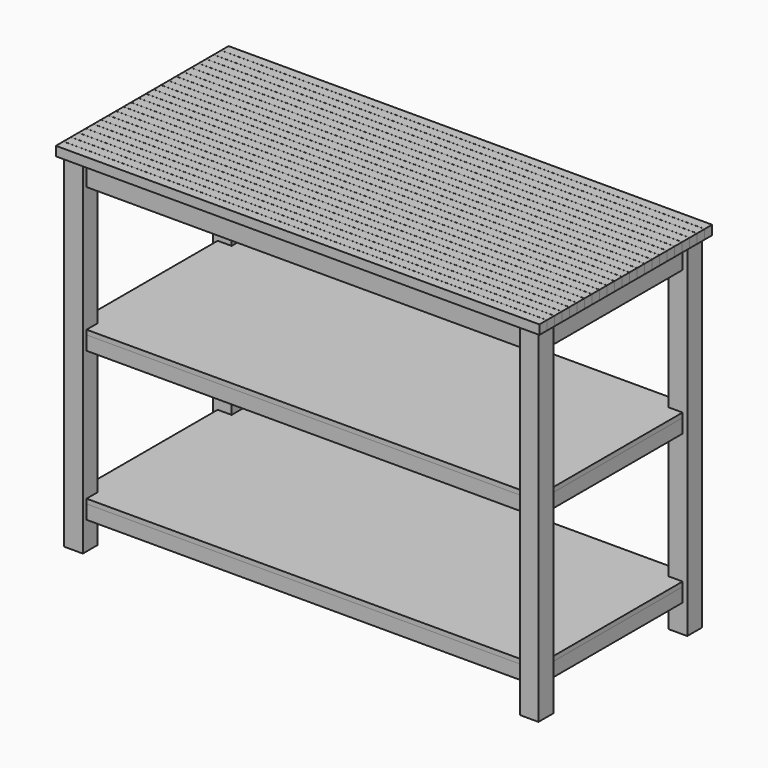
from build123d import *

# Parameters (mm, degrees)
F0_W      = 50.8
F0_H      = 50.8
F1_DEPTH  = 939.8
F2_W      = 1193.8
F2_H      = 25.4
F3_DEPTH  = 63.5
F2_W_2    = 25.4
F2_H_2    = 457.2
F5_W      = 1270
F5_H      = 533.4
F5_W_2    = 1219.2
F5_H_2    = 482.6
F6_DEPTH  = 38.1
F7_W      = 1270
F7_H      = 533.4
F8_DEPTH  = 12.7
F10_W     = 1270
F10_H     = 533.4
F10_W_2   = 1219.2
F10_H_2   = 482.6
F11_DEPTH = 38.1
F13_W     = 1320.8
F13_H     = 25.4
F14_DEPTH = 25.4
F12_W     = 1219.2
F12_H     = 482.6
F15_DEPTH = 12.7


# Not quite as in the source:
# - ends of sketch curves that miss each other by under 0.0002 mm in the source are joined


with BuildPart() as f1:
    # F0 (on Top) → F1 (new body)
    with BuildSketch(Plane.XY):
        with Locations((25.4, 25.4)):
            Rectangle(F0_W, F0_H)
    extrude(amount=F1_DEPTH)


with BuildPart() as f1b:
    # F0 (on Top) → F1, piece 2 (new body)
    with BuildSketch(Plane.XY):
        with Locations((25.4, 533.4)):
            Rectangle(F0_W, F0_H)
    extrude(amount=F1_DEPTH)


with BuildPart() as f1c:
    # F0 (on Top) → F1, piece 3 (new body)
    with BuildSketch(Plane.XY):
        with Locations((1270, 25.4)):
            Rectangle(F0_W, F0_H)
    extrude(amount=F1_DEPTH)


with BuildPart() as f1d:
    # F0 (on Top) → F1, piece 4 (new body)
    with BuildSketch(Plane.XY):
        with Locations((1270, 533.4)):
            Rectangle(F0_W, F0_H)
    extrude(amount=F1_DEPTH)


with BuildPart() as f3:
    # F2 (on face) → F3 (new body)
    with BuildSketch(Plane.XY.offset(939.8)):
        with Locations((647.7, 533.4)):
            Rectangle(F2_W, F2_H)
    extrude(amount=-F3_DEPTH)


with BuildPart() as f3b:
    # F2 (on face) → F3, piece 2 (new body)
    with BuildSketch(Plane.XY.offset(939.8)):
        with Locations((647.7, 25.4)):
            Rectangle(F2_W, F2_H)
    extrude(amount=-F3_DEPTH)


with BuildPart() as f3c:
    # F2 (on face) → F3, piece 3 (new body)
    with BuildSketch(Plane.XY.offset(939.8)):
        with Locations((25.4, 279.4)):
            Rectangle(F2_W_2, F2_H_2)
    extrude(amount=-F3_DEPTH)


with BuildPart() as f3d:
    # F2 (on face) → F3, piece 4 (new body)
    with BuildSketch(Plane.XY.offset(939.8)):
        with Locations((1270, 279.4)):
            Rectangle(F2_W_2, F2_H_2)
    extrude(amount=-F3_DEPTH)


with BuildPart() as f6:
    # F5 (on offset) → F6 (new body)
    with BuildSketch(Plane.XY.offset(76.2)):
        with Locations((647.7, 279.4)):
            Rectangle(F5_W, F5_H)
        with Locations((647.7, 279.4)):
            Rectangle(F5_W_2, F5_H_2, mode=Mode.SUBTRACT)
    extrude(amount=F6_DEPTH)


with BuildPart() as f8:
    # F7 (on face) → F8 (new body)
    with BuildSketch(Plane.XY.offset(114.3)):
        with Locations((647.7, 279.4)):
            Rectangle(F7_W, F7_H)
    extrude(amount=F8_DEPTH)


with BuildPart() as f11:
    # F10 (on offset) → F11 (new body)
    with BuildSketch(Plane.XY.offset(520.7)):
        with Locations((647.7, 279.4)):
            Rectangle(F10_W, F10_H)
        with Locations((647.7, 279.4)):
            Rectangle(F10_W_2, F10_H_2, mode=Mode.SUBTRACT)
    extrude(amount=-F11_DEPTH)


with BuildPart() as f14:
    # F13 (on face) → F14 (new body)
    with BuildSketch(Plane.XY.offset(939.8)):
        with Locations((647.7, 0)):
            Rectangle(F13_W, F13_H)
    extrude(amount=F14_DEPTH)


with BuildPart() as f14b:
    # F13 (on face) → F14, piece 2 (new body)
    with BuildSketch(Plane.XY.offset(939.8)):
        with Locations((647.7, 25.654)):
            Rectangle(F13_W, F13_H)
    extrude(amount=F14_DEPTH)


with BuildPart() as f14c:
    # F13 (on face) → F14, piece 3 (new body)
    with BuildSketch(Plane.XY.offset(939.8)):
        with Locations((647.7, 51.308)):
            Rectangle(F13_W, F13_H)
    extrude(amount=F14_DEPTH)


with BuildPart() as f14d:
    # F13 (on face) → F14, piece 4 (new body)
    with BuildSketch(Plane.XY.offset(939.8)):
        with Locations((647.7, 76.962)):
            Rectangle(F13_W, F13_H)
    extrude(amount=F14_DEPTH)


with BuildPart() as f14e:
    # F13 (on face) → F14, piece 5 (new body)
    with BuildSketch(Plane.XY.offset(939.8)):
        with Locations((647.7, 102.616)):
            Rectangle(F13_W, F13_H)
    extrude(amount=F14_DEPTH)


with BuildPart() as f14f:
    # F13 (on face) → F14, piece 6 (new body)
    with BuildSketch(Plane.XY.offset(939.8)):
        with Locations((647.7, 128.27)):
            Rectangle(F13_W, F13_H)
    extrude(amount=F14_DEPTH)


with BuildPart() as f14g:
    # F13 (on face) → F14, piece 7 (new body)
    with BuildSketch(Plane.XY.offset(939.8)):
        with Locations((647.7, 153.924)):
            Rectangle(F13_W, F13_H)
    extrude(amount=F14_DEPTH)


with BuildPart() as f14h:
    # F13 (on face) → F14, piece 8 (new body)
    with BuildSketch(Plane.XY.offset(939.8)):
        with Locations((647.7, 179.578)):
            Rectangle(F13_W, F13_H)
    extrude(amount=F14_DEPTH)


with BuildPart() as f14i:
    # F13 (on face) → F14, piece 9 (new body)
    with BuildSketch(Plane.XY.offset(939.8)):
        with Locations((647.7, 205.232)):
            Rectangle(F13_W, F13_H)
    extrude(amount=F14_DEPTH)


with BuildPart() as f14j:
    # F13 (on face) → F14, piece 10 (new body)
    with BuildSketch(Plane.XY.offset(939.8)):
        with Locations((647.7, 230.886)):
            Rectangle(F13_W, F13_H)
    extrude(amount=F14_DEPTH)


with BuildPart() as f14k:
    # F13 (on face) → F14, piece 11 (new body)
    with BuildSketch(Plane.XY.offset(939.8)):
        with Locations((647.7, 256.54)):
            Rectangle(F13_W, F13_H)
    extrude(amount=F14_DEPTH)


with BuildPart() as f14l:
    # F13 (on face) → F14, piece 12 (new body)
    with BuildSketch(Plane.XY.offset(939.8)):
        with Locations((647.7, 282.194)):
            Rectangle(F13_W, F13_H)
    extrude(amount=F14_DEPTH)


with BuildPart() as f14m:
    # F13 (on face) → F14, piece 13 (new body)
    with BuildSketch(Plane.XY.offset(939.8)):
        with Locations((647.7, 307.848)):
            Rectangle(F13_W, F13_H)
    extrude(amount=F14_DEPTH)


with BuildPart() as f14n:
    # F13 (on face) → F14, piece 14 (new body)
    with BuildSketch(Plane.XY.offset(939.8)):
        with Locations((647.7, 333.502)):
            Rectangle(F13_W, F13_H)
    extrude(amount=F14_DEPTH)


with BuildPart() as f14o:
    # F13 (on face) → F14, piece 15 (new body)
    with BuildSketch(Plane.XY.offset(939.8)):
        with Locations((647.7, 359.156)):
            Rectangle(F13_W, F13_H)
    extrude(amount=F14_DEPTH)


with BuildPart() as f14p:
    # F13 (on face) → F14, piece 16 (new body)
    with BuildSketch(Plane.XY.offset(939.8)):
        with Locations((647.7, 384.81)):
            Rectangle(F13_W, F13_H)
    extrude(amount=F14_DEPTH)


with BuildPart() as f14q:
    # F13 (on face) → F14, piece 17 (new body)
    with BuildSketch(Plane.XY.offset(939.8)):
        with Locations((647.7, 410.464)):
            Rectangle(F13_W, F13_H)
    extrude(amount=F14_DEPTH)


with BuildPart() as f14r:
    # F13 (on face) → F14, piece 18 (new body)
    with BuildSketch(Plane.XY.offset(939.8)):
        with Locations((647.7, 436.118)):
            Rectangle(F13_W, F13_H)
    extrude(amount=F14_DEPTH)


with BuildPart() as f14s:
    # F13 (on face) → F14, piece 19 (new body)
    with BuildSketch(Plane.XY.offset(939.8)):
        with Locations((647.7, 461.772)):
            Rectangle(F13_W, F13_H)
    extrude(amount=F14_DEPTH)


with BuildPart() as f14t:
    # F13 (on face) → F14, piece 20 (new body)
    with BuildSketch(Plane.XY.offset(939.8)):
        with Locations((647.7, 487.426)):
            Rectangle(F13_W, F13_H)
    extrude(amount=F14_DEPTH)


with BuildPart() as f14u:
    # F13 (on face) → F14, piece 21 (new body)
    with BuildSketch(Plane.XY.offset(939.8)):
        with Locations((647.7, 513.08)):
            Rectangle(F13_W, F13_H)
    extrude(amount=F14_DEPTH)


with BuildPart() as f14v:
    # F13 (on face) → F14, piece 22 (new body)
    with BuildSketch(Plane.XY.offset(939.8)):
        with Locations((647.7, 538.734)):
            Rectangle(F13_W, F13_H)
    extrude(amount=F14_DEPTH)


with BuildPart() as f14w:
    # F13 (on face) → F14, piece 23 (new body)
    with BuildSketch(Plane.XY.offset(939.8)):
        with Locations((647.7, 564.388)):
            Rectangle(F13_W, F13_H)
    extrude(amount=F14_DEPTH)


with BuildPart() as f15:
    # F12 (on face) → F15 (new body)
    with BuildSketch(Plane.XY.offset(520.7)):
        Polygon((1282.7, 546.1), (12.6999995756, 546.1), (12.7, 12.7), (1282.5777116191, 12.7), (1282.7, 12.7), align=None)
        with Locations((647.7, 279.4)):
            Rectangle(F12_W, F12_H, mode=Mode.SUBTRACT)
        with Locations((647.7, 279.4)):
            Rectangle(F12_W, F12_H)
    extrude(amount=F15_DEPTH)


solid = Compound([f1.part, f1b.part, f1c.part, f1d.part, f3.part, f3b.part, f3c.part, f3d.part, f6.part, f8.part, f11.part, f14.part, f14b.part, f14c.part, f14d.part, f14e.part, f14f.part, f14g.part, f14h.part, f14i.part, f14j.part, f14k.part, f14l.part, f14m.part, f14n.part, f14o.part, f14p.part, f14q.part, f14r.part, f14s.part, f14t.part, f14u.part, f14v.part, f14w.part, f15.part])
